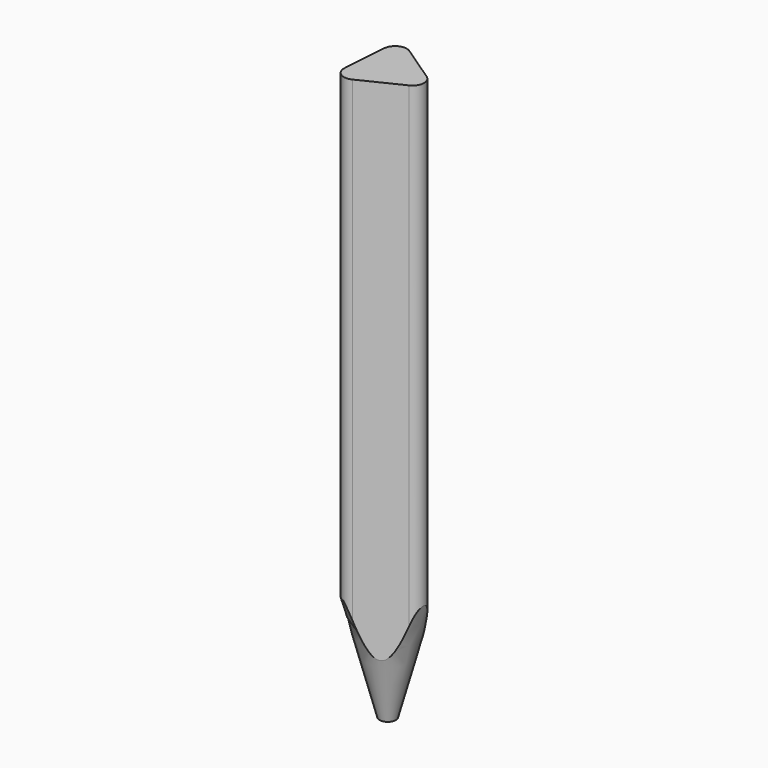
from build123d import *

# Parameters (mm, degrees)
F0_R                   = 18.8444489445
F1_DEPTH               = 74.676
DRAFT_F1_DRAFTED_ANGLE = 15
F2_DEPTH               = 57.15
F3_DEPTH               = 191.262


# Not quite as in the source:
# - an extrude with a draft is written as a straight extrude whose walls are then drafted


with BuildPart() as f1:
    # F0 (on Top) → F1 (new body)
    with BuildSketch(Plane.XY):
        Circle(F0_R)
        with BuildLine():
            ThreePointArc((-10.0701897307, 10.6265741961), (-7.227449582, 14.8367082138), (-2.159996495, 14.4798900375))
            Line((-2.159996495, 14.4798900375), (14.2379780744, 3.4077530297))
            ThreePointArc((14.2379780744, 3.4077530297), (16.4626910127, -1.1591991643), (13.619950864, -5.369333182))
            Line((13.619950864, -5.369333182), (-4.1677883437, -14.0343272258))
            ThreePointArc((-4.1677883437, -14.0343272258), (-9.2352414307, -13.6775090495), (-11.459954369, -9.1105568555))
            Line((-11.459954369, -9.1105568555), (-10.0701897307, 10.6265741961))
        make_face(mode=Mode.SUBTRACT)
        with BuildLine():
            Line((14.2379780744, 3.4077530297), (-2.159996495, 14.4798900375))
            ThreePointArc((-2.159996495, 14.4798900375), (-7.227449582, 14.8367082138), (-10.0701897307, 10.6265741961))
            Line((-10.0701897307, 10.6265741961), (-11.459954369, -9.1105568555))
            ThreePointArc((-11.459954369, -9.1105568555), (-9.2352414307, -13.6775090495), (-4.1677883437, -14.0343272258))
            Line((-4.1677883437, -14.0343272258), (13.619950864, -5.369333182))
            ThreePointArc((13.619950864, -5.369333182), (16.4626910127, -1.1591991643), (14.2379780744, 3.4077530297))
        make_face()
    extrude(amount=-F1_DEPTH)

    # draft_F1_drafted
    draft_f1_drafted_walls = [f1.faces().sort_by_distance(p)[0] for p in [
        (-18.8444489445, 0, -49.784),
    ]]
    draft(draft_f1_drafted_walls, neutral_plane=Plane(origin=(0, 0, 0), x_dir=(1, 0, 0), z_dir=(0, 0, -1)), angle=DRAFT_F1_DRAFTED_ANGLE)

    # F0 (on Top) → F2 (intersect)
    with BuildSketch(Plane.XY):
        with BuildLine():
            Line((14.2379780744, 3.4077530297), (-2.159996495, 14.4798900375))
            ThreePointArc((-2.159996495, 14.4798900375), (-7.227449582, 14.8367082138), (-10.0701897307, 10.6265741961))
            Line((-10.0701897307, 10.6265741961), (-11.459954369, -9.1105568555))
            ThreePointArc((-11.459954369, -9.1105568555), (-9.2352414307, -13.6775090495), (-4.1677883437, -14.0343272258))
            Line((-4.1677883437, -14.0343272258), (13.619950864, -5.369333182))
            ThreePointArc((13.619950864, -5.369333182), (16.4626910127, -1.1591991643), (14.2379780744, 3.4077530297))
        make_face()
    extrude(amount=-F2_DEPTH, mode=Mode.INTERSECT)

    # F0 (on Top) → F3 (join)
    with BuildSketch(Plane.XY):
        with BuildLine():
            Line((14.2379780744, 3.4077530297), (-2.159996495, 14.4798900375))
            ThreePointArc((-2.159996495, 14.4798900375), (-7.227449582, 14.8367082138), (-10.0701897307, 10.6265741961))
            Line((-10.0701897307, 10.6265741961), (-11.459954369, -9.1105568555))
            ThreePointArc((-11.459954369, -9.1105568555), (-9.2352414307, -13.6775090495), (-4.1677883437, -14.0343272258))
            Line((-4.1677883437, -14.0343272258), (13.619950864, -5.369333182))
            ThreePointArc((13.619950864, -5.369333182), (16.4626910127, -1.1591991643), (14.2379780744, 3.4077530297))
        make_face()
    extrude(amount=F3_DEPTH)


solid = f1.part
